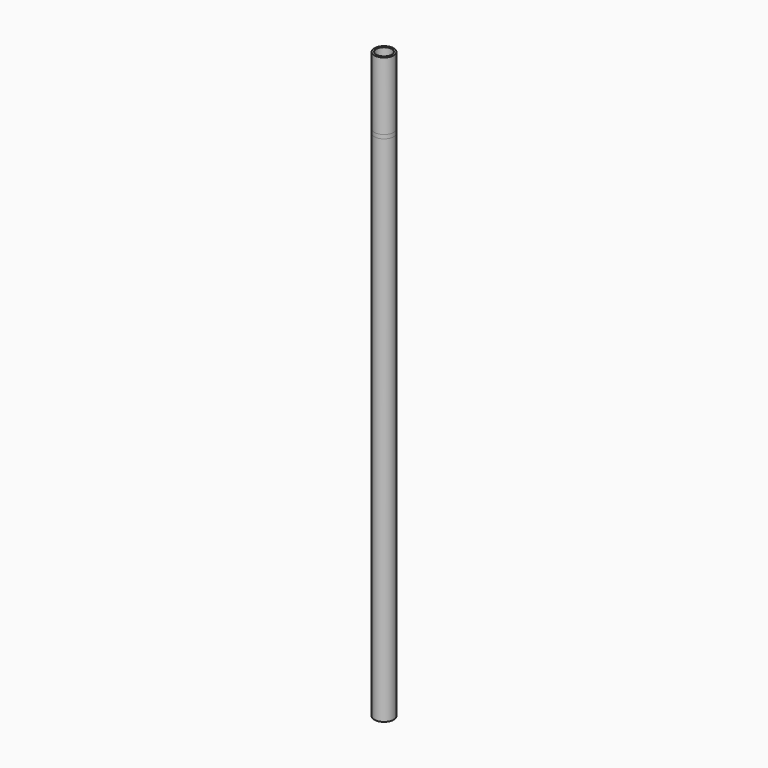
from build123d import *

# Parameters (mm, degrees)
F0_R     = 3.99
F0_R_2   = 2
F1_DEPTH = 14
F2_R     = 2
F3_DEPTH = 11.2
F0_R_3   = 5
F4_DEPTH = 2
F5_DEPTH = 12
F6_DEPTH = 35
F7_DEPTH = 265


# Not quite as in the source:
# - a feature names something its author has since deleted; it is built from what else it names


with BuildPart() as f1:
    # F0 (on Top) → F1 (new body)
    with BuildSketch(Plane.XY):
        Circle(F0_R)
        Circle(F0_R_2, mode=Mode.SUBTRACT)
    extrude(amount=F1_DEPTH)

    # F2 (on face) → F3 (cut)
    with BuildSketch(Plane.XY.offset(14)):
        with BuildLine():
            ThreePointArc((-2.1, 3.3926538285), (0, 3.99), (2.1, 3.3926538285))
            Line((2.1, 3.3926538285), (2.1, 5))
            Line((2.1, 5), (-2.1, 5))
            Line((-2.1, 5), (-2.1, 3.3926538285))
        make_face()
        with BuildLine():
            Line((2.1, -3.3926538285), (2.1, 3.3926538285))
            ThreePointArc((2.1, 3.3926538285), (0, 3.99), (-2.1, 3.3926538285))
            Line((-2.1, 3.3926538285), (-2.1, -3.3926538285))
            ThreePointArc((-2.1, -3.3926538285), (0, -3.99), (2.1, -3.3926538285))
        make_face()
        Circle(F2_R, mode=Mode.SUBTRACT)
        with BuildLine():
            Line((2.1, -5), (2.1, -3.3926538285))
            ThreePointArc((2.1, -3.3926538285), (0, -3.99), (-2.1, -3.3926538285))
            Line((-2.1, -3.3926538285), (-2.1, -5))
            Line((-2.1, -5), (2.1, -5))
        make_face()
    extrude(amount=-F3_DEPTH, mode=Mode.SUBTRACT)

    # F0 (on Top) → F4 (join)
    with BuildSketch(Plane.XY):
        Circle(F0_R_3)
        Circle(F0_R, mode=Mode.SUBTRACT)
    extrude(amount=F4_DEPTH)

    # F0 (on Top) → F5 (join)
    with BuildSketch(Plane.XY):
        Circle(F0_R)
        Circle(F0_R_2, mode=Mode.SUBTRACT)
    extrude(amount=-F5_DEPTH)


with BuildPart() as f6:
    # F6 (new): a face of the model
    f6_faces = [f1.part.faces().sort_by_distance(p)[0] for p in [
        (-4.8585786438, 0, 2),
    ]]
    extrude(f6_faces, amount=F6_DEPTH)


with BuildPart() as f7:
    # F7 (new): a face of the model
    f7_faces = [f1.part.faces().sort_by_distance(p)[0] for p in [
        (-4.8585786438, 0, 0),
    ]]
    extrude(f7_faces, amount=F7_DEPTH)


solid = Compound([f1.part, f6.part, f7.part])
